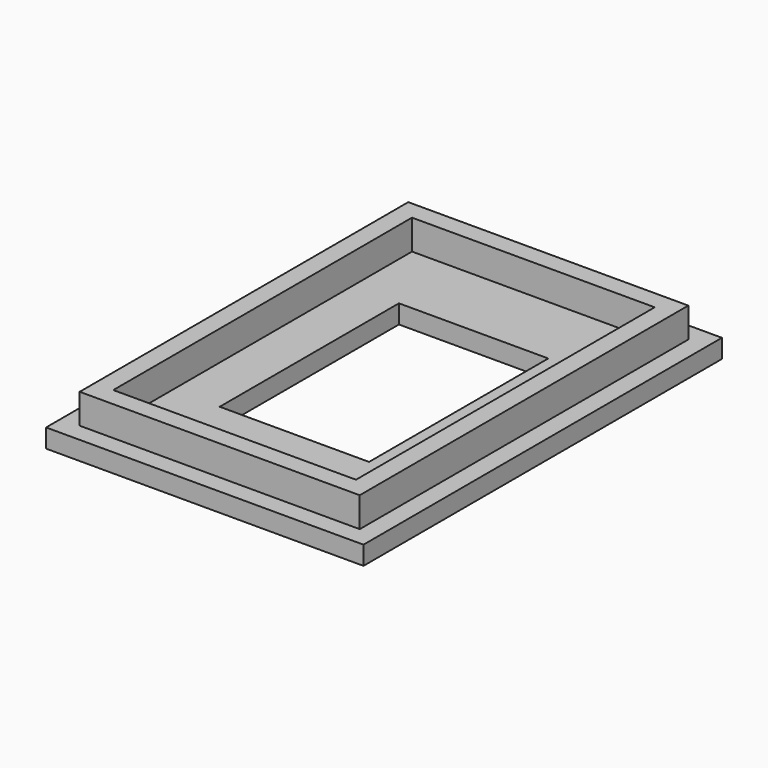
from build123d import *

# Parameters (mm, degrees)
F0_W        = 53.975
F0_H        = 76.2
F1_DEPTH    = 3.175
F2_W        = 47.625
F2_H        = 69.85
F3_DEPTH    = 5.08
F4_T        = 3.175
F4_T3_DEPTH = 53.975
F4_T5_DEPTH = 76.2
F5_W        = 25.4
F5_H        = 38.1
F6_DEPTH    = 25.4


# Not quite as in the source:
# - a shell that OpenCascade refuses in one call is made with other operations: the cavity is built on its own and cut out


with BuildPart() as f1:
    # F0 (on Top) → F1 (new body)
    with BuildSketch(Plane.XY):
        Rectangle(F0_W, F0_H)
    extrude(amount=F1_DEPTH)

    # F2 (on face) → F3 (join)
    with BuildSketch(Plane.XY.offset(3.175)):
        Rectangle(F2_W, F2_H)
    extrude(amount=F3_DEPTH)

    # F4: shell of thickness 3.175, made by hand


with BuildPart() as f4_core1:
    # F4_t2: copy of F1
    add(f1.part)

    # the walls: a layer under each face that stays
    f4_faces = [f4_core1.faces().sort_by_distance(p)[0] for p in [
        (0, 38.1, 1.5875),
        (26.9875, 0, 1.5875),
        (-26.9875, 0, 1.5875),
        (0, 0, 0),
        (-25.1883333333, -35.56, 3.175),
        (0, -38.1, 1.5875),
        (0, 34.925, 5.715),
        (-23.8125, 0, 5.715),
        (0, -34.925, 5.715),
        (23.8125, 0, 5.715),
    ]]
    thicken(f4_faces, amount=-F4_T, mode=Mode.SUBTRACT)

    # F4_s4 → F4_t3 (cut)
    with BuildSketch(Plane.YZ.offset(-26.9875)):
        Polygon((34.95675, 3.20675), (34.925, 0), (31.75, 0), (31.75, 3.175), align=None)
        Polygon((-34.95675, 3.20675), (-34.925, 0), (-31.75, 0), (-31.75, 3.175), align=None)
    extrude(amount=F4_T3_DEPTH, mode=Mode.SUBTRACT)

    # F4_s6 → F4_t5 (cut)
    with BuildSketch(Plane.XZ.offset(-38.1)):
        Polygon((-23.84425, 3.20675), (-23.8125, 0), (-20.6375, 0), (-20.6375, 3.175), align=None)
        Polygon((23.84425, 3.20675), (23.8125, 0), (20.6375, 0), (20.6375, 3.175), align=None)
    extrude(amount=F4_T5_DEPTH, mode=Mode.SUBTRACT)


with BuildPart() as f1_1:
    add(f1.part)

    # what is left inside the walls is the cavity
    f4_cavity = [f4_core1.part.solids().sort_by_distance(p)[0] for p in [
        (0, -10.583333, 3.20675),
    ]]
    add(f4_cavity, mode=Mode.SUBTRACT)

    # F5 (on face) → F6 (cut)
    with BuildSketch(Plane.XY.offset(3.175)):
        Rectangle(F5_W, F5_H)
    extrude(amount=-F6_DEPTH, mode=Mode.SUBTRACT)


solid = f1_1.part
